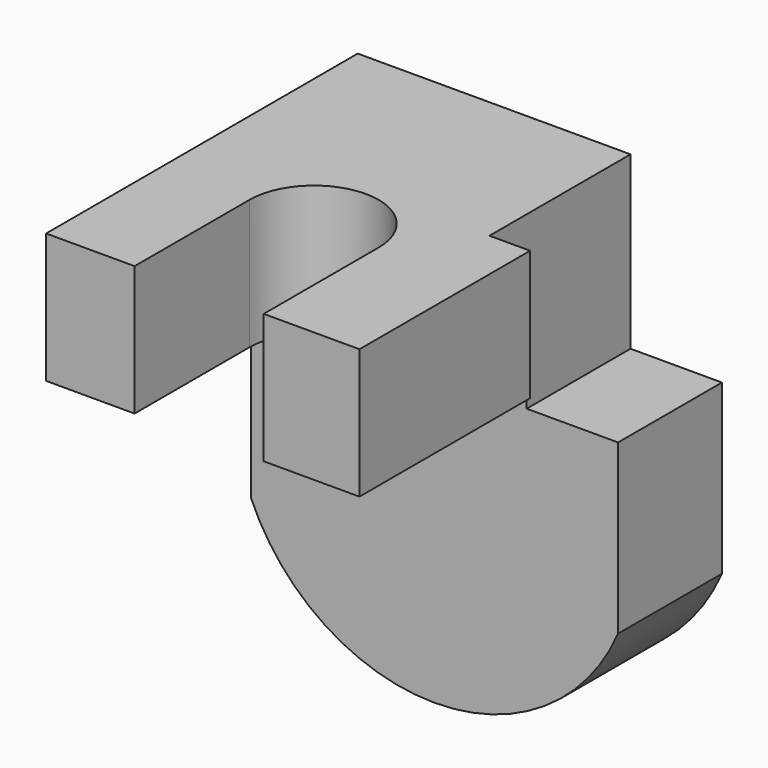
from build123d import *

# Parameters (mm, degrees)
F1_DEPTH = 25.4
F3_DEPTH = 25.4


# Not quite as in the source:
# - ends of sketch curves that miss each other by under 0.0002 mm in the source are joined


with BuildPart() as f1:
    # F0 (on Front) → F1 (new body)
    with BuildSketch(Plane.XZ):
        with BuildLine():
            Line((0, 0), (-53.9480485022, 0))
            Line((-53.9480485022, 0), (-53.9480485022, -41.0289131105))
            ThreePointArc((-53.9480485022, -41.0289131105), (-18.0300064385, -64.6250791293), (17.8880356252, -41.0289131105))
            Line((17.8880356252, -41.0289131105), (17.8880356252, -8.0922106281))
            Line((17.8880356252, -8.0922106281), (0, -8.0922106281))
            Line((0, -8.0922106281), (0, 0))
        make_face()
    extrude(amount=F1_DEPTH)

    # F2 (on Top) → F3 (join)
    with BuildSketch(Plane.XY):
        with BuildLine():
            Line((0, -34.4983525574), (0, -25.6963036954))
            Line((0, -25.6963036954), (0, 0))
            Line((0, 0), (-53.380176425, 0))
            Line((-53.380176425, 0), (-53.380176425, -25.9802397341))
            Line((-53.380176425, -25.9802397341), (-53.380176425, -76.2371048331))
            Line((-53.380176425, -76.2371048331), (-36.0600091517, -76.2371048331))
            Line((-36.0600091517, -76.2371048331), (-36.0600091517, -48.1273345649))
            ThreePointArc((-36.0600091517, -48.1273345649), (-23.424807936, -35.4921333492), (-10.7896067202, -48.1273345649))
            Line((-10.7896067202, -48.1273345649), (-10.7896067202, -76.2371048331))
            Line((-10.7896067202, -76.2371048331), (7.9502388835, -76.2371048331))
            Line((7.9502388835, -76.2371048331), (7.9502388835, -34.4983525574))
            Line((7.9502388835, -34.4983525574), (0, -34.4983525574))
        make_face()
    extrude(amount=F3_DEPTH)


solid = f1.part
